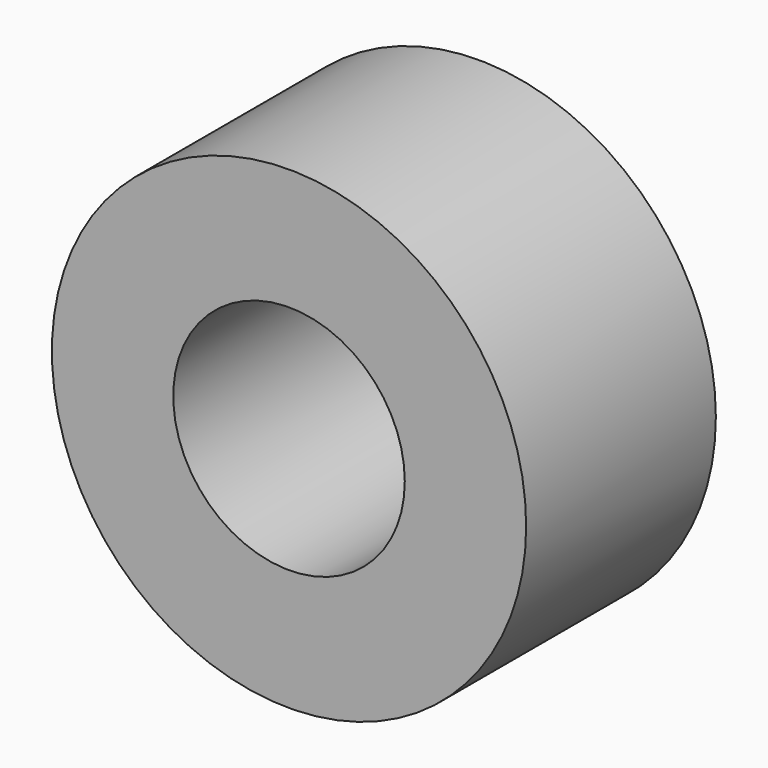
from build123d import *

# Parameters (mm, degrees)
F0_R     = 3.175
F0_R_2   = 1.55
F1_DEPTH = 3.175


# Not quite as in the source:
# - a length typed as a fraction of an inch, garbled in the dataset ("3 / 203.2 mm" for 3/8 in), is restored


with BuildPart() as f1:
    # F0 (on Front) → F1 (new body)
    with BuildSketch(Plane.XZ):
        Circle(F0_R)
        Circle(F0_R_2, mode=Mode.SUBTRACT)
    extrude(amount=F1_DEPTH)


solid = f1.part
